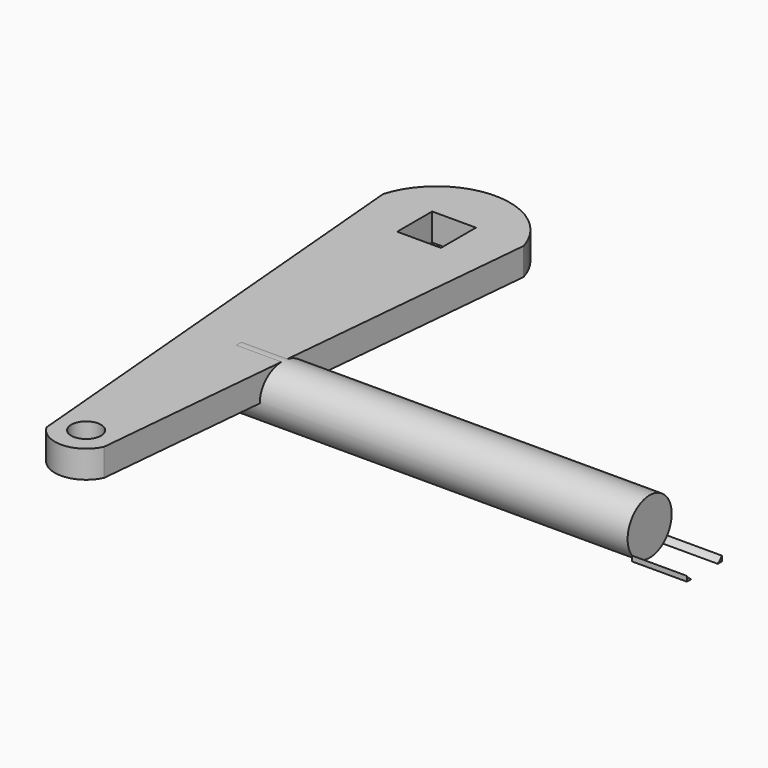
from build123d import *

# Parameters (mm, degrees)
F0_R     = 5.0345603454
F1_DEPTH = 75
F3_W     = 8
F3_H     = 8
F4_DEPTH = 5
F6_DEPTH = 10
F7_R     = 2.7283514887
F8_DEPTH = 25


with BuildPart() as f1:
    # F0 (on Right) → F1 (new body)
    with BuildSketch(Plane.YZ):
        Circle(F0_R)
    extrude(amount=F1_DEPTH)

    # F3 (on Top) → F4 (join)
    with BuildSketch(Plane.XY):
        with BuildLine():
            add(Edge.make_bspline(
                [(12.8348679437, 48.9545158337), (10.1793770282, 20.3342274985), (7.5238861127, -8.231182894), (4.8683951972, -36.8514712291)],
                knots=[0, 0, 0, 0, 86.1750085805, 86.1750085805, 86.1750085805, 86.1750085805], degree=3))
            ThreePointArc((12.8348679437, 48.9545158337), (-2.794e-06, 58.504055005), (-12.8348735316, 48.9545158337))
            add(Edge.make_bspline(
                [(-12.8348735316, 48.9545158337), (-10.3269097443, 20.1867005239), (-7.8189459569, -8.5262368434), (-5.3109821696, -37.2940521532)],
                knots=[0, 0, 0, 0, 86.5761192305, 86.5761192305, 86.5761192305, 86.5761192305], degree=3))
            ThreePointArc((-5.3109821696, -37.2940521532), (-0.0857201671, -40.1909529666), (4.8683951972, -36.8514712291))
        make_face()
        with Locations((-2.794e-06, 45.1040573379)):
            Rectangle(F3_W, F3_H, mode=Mode.SUBTRACT)
    extrude(amount=F4_DEPTH)

    # F7 (on face) → F8 (cut)
    with BuildSketch(Plane.XY.offset(5)):
        with Locations((-0.3341082492, -34.4780180346)):
            Circle(F7_R)
    extrude(amount=-F8_DEPTH, mode=Mode.SUBTRACT)


with BuildPart() as f6:
    # F5 (on face) → F6 (new body)
    with BuildSketch(Plane.YZ.offset(75)):
        with BuildLine():
            Line((3.0572533215, -4), (4, -4))
            Line((4, -4), (4, -3.0572533215))
            ThreePointArc((4, -3.0572533215), (3.5599717605, -3.5599717605), (3.0572533215, -4))
        make_face()
    extrude(amount=F6_DEPTH)


with BuildPart() as f6b:
    # F5 (on face) → F6, piece 2 (new body)
    with BuildSketch(Plane.YZ.offset(75)):
        with BuildLine():
            Line((-4, -4), (-3.0572533215, -4))
            ThreePointArc((-3.0572533215, -4), (-3.5599717605, -3.5599717605), (-4, -3.0572533215))
            Line((-4, -3.0572533215), (-4, -4))
        make_face()
    extrude(amount=F6_DEPTH)


solid = Compound([f1.part, f6.part, f6b.part])
